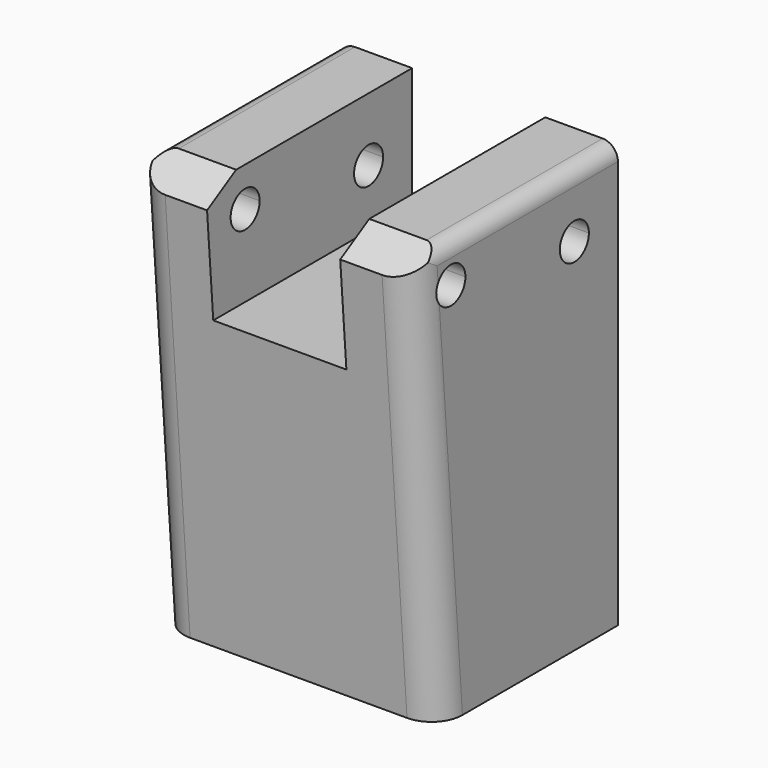
from build123d import *

# Parameters (mm, degrees)
F1_DEPTH     = 46
F3_DEPTH     = 40
F5_DEPTH     = 254
F6_W         = 22
F6_H         = 20
F7_DEPTH     = 1346.2
F8_DEPTH     = 65
F10_DEPTH    = 127
F12_DEPTH    = 254
F14_DEPTH    = 254
F15_T1_DEPTH = 103.8636030304
F15_T3_DEPTH = 103.8636030304
F17_T1_DEPTH = 49.0578822911


# Not quite as in the source:
# - a fillet or chamfer that OpenCascade refuses, or shapes differently, is made with other operations: its cross-section is extruded or revolved along the edge and cut away or added
# - a feature of the source that left no trace in its solid (it failed there, or was rolled back) is left out


with BuildPart() as f1:
    # F0 (on Right) → F1 (new body)
    with BuildSketch(Plane.YZ):
        Polygon((52, 0), (0, 0), (12, -60), (12, -70), (52, -70), align=None)
    extrude(amount=F1_DEPTH)

    # F2 (on face) → F3 (cut)
    with BuildSketch(Plane(origin=(0, 0, -70), x_dir=(1, 0, 0), z_dir=(0, 0, -1))):
        with BuildLine():
            Line((23, -33.3181476), (38, -33.3181476))
            ThreePointArc((38, -33.3181476), (12.3933982822, -22.7115458822), (23, -48.3181476))
            Line((23, -48.3181476), (23, -33.3181476))
        make_face()
        with BuildLine():
            ThreePointArc((23, -48.3181476), (33.6066017178, -43.9247493178), (38, -33.3181476))
            Line((38, -33.3181476), (23, -33.3181476))
            Line((23, -33.3181476), (23, -48.3181476))
        make_face()
    extrude(amount=-F3_DEPTH, mode=Mode.SUBTRACT)

    # F4 (on face) → F5 (cut)
    with BuildSketch(Plane.YZ.offset(46)):
        with BuildLine():
            Line((17.5, -6.5), (20.5, -6.5))
            ThreePointArc((20.5, -6.5), (19.6213203436, -4.3786796564), (17.5, -3.5))
            Line((17.5, -3.5), (17.5, -6.5))
        make_face()
        with BuildLine():
            ThreePointArc((17.5, -3.5), (15.3786796564, -8.6213203436), (20.5, -6.5))
            Line((20.5, -6.5), (17.5, -6.5))
            Line((17.5, -6.5), (17.5, -3.5))
        make_face()
    extrude(amount=-F5_DEPTH, mode=Mode.SUBTRACT)

    # F6 (on face) → F7 (cut)
    with BuildSketch(Plane(origin=(0, 52, 0), x_dir=(-1, 0, 0), z_dir=(0, 1, 0))):
        with Locations((-23, -10)):
            Rectangle(F6_W, F6_H)
    extrude(amount=-F7_DEPTH, mode=Mode.SUBTRACT)

    # F4 (on face) → F8 (cut)
    with BuildSketch(Plane.YZ.offset(46)):
        with BuildLine():
            ThreePointArc((43, -7.5), (40.8786796564, -12.6213203436), (46, -10.5))
            ThreePointArc((46, -10.5), (45.1213203436, -8.3786796564), (43, -7.5))
        make_face()
    extrude(amount=-F8_DEPTH, mode=Mode.SUBTRACT)

    # F9 (on face) → F10 (cut)
    with BuildSketch(Plane.YZ.offset(46)):
        Polygon((1.1435132474, -8.0939428881), (1.6304426827, -8.0939428881), (15.6421177089, 0), (0, 0), align=None)
    extrude(amount=-F10_DEPTH, mode=Mode.SUBTRACT)

    # F11 (on Right) → F12 (cut)
    with BuildSketch(Plane.YZ):
        Polygon((0, -70.3560113907), (14.7977182642, -70.0814500451), (9.3696815893, 0), (0, 0), align=None)
    extrude(amount=F12_DEPTH, mode=Mode.SUBTRACT)

    # F13 (on face) → F14 (cut)
    with BuildSketch(Plane.XY):
        with BuildLine():
            add(Edge.make_bspline(
                [(0, 12.6551715657), (0, 9.9420361221), (2.5992305018, 9.7406599671), (3.9225574583, 9.6255876124)],
                knots=[0, 0, 0, 0, 4.9562925603, 4.9562925603, 4.9562925603, 4.9562925603], degree=3))
            Line((0, 12.6551715657), (0, 9.539283812))
            Line((0, 9.539283812), (3.9225574583, 9.6255876124))
        make_face()
        with BuildLine():
            Line((46, 9.539283812), (46, 12.6551715657))
            add(Edge.make_bspline(
                [(46, 12.6551715657), (46, 9.9420361221), (43.4007694982, 9.7406599671), (42.0774425417, 9.6255876124)],
                knots=[0, 0, 0, 0, 4.9562925603, 4.9562925603, 4.9562925603, 4.9562925603], degree=3))
            Line((42.0774425417, 9.6255876124), (46, 9.539283812))
        make_face()
    extrude(amount=-F14_DEPTH, mode=Mode.SUBTRACT)

    # F15: fillet of radius 5.08 on 2 edges, made by hand

    # F15_s2 → F15_t1 (cut)
    with BuildSketch(Plane(origin=(0, 6.4583208178, -83.3834616235), x_dir=(1, 0, 0), z_dir=(0, -0.0772219774, 0.9970139248))):
        with BuildLine():
            ThreePointArc((0, 14.4217030153), (1.4878975516, 10.8296005669), (5.08, 9.3417030153))
            Line((5.08, 9.3417030153), (0, 9.3417030153))
            Line((0, 9.3417030153), (0, 14.4217030153))
        make_face()
    extrude(amount=F15_T1_DEPTH, mode=Mode.SUBTRACT)

    # F15_s4 → F15_t3 (cut)
    with BuildSketch(Plane(origin=(0, -1.5622319844, 20.169996876), x_dir=(1, 0, 0), z_dir=(0, 0.0772219774, -0.9970139248))):
        with BuildLine():
            ThreePointArc((40.92, -9.3417030153), (44.5121024484, -10.8296005669), (46, -14.4217030153))
            Line((46, -14.4217030153), (46, -9.3417030153))
            Line((46, -9.3417030153), (40.92, -9.3417030153))
        make_face()
    extrude(amount=F15_T3_DEPTH, mode=Mode.SUBTRACT)

    # F17: fillet of radius 2.54 on 2 edges, made by hand

    # F17_s2 → F17_t1 (cut)
    with BuildSketch(Plane.XZ.offset(-58.35)):
        with BuildLine():
            ThreePointArc((2.54, 0), (0.7439487758, -0.7439487758), (0, -2.54))
            Line((0, -2.54), (0, 0))
            Line((0, 0), (2.54, 0))
        make_face()
        with BuildLine():
            ThreePointArc((43.46, 0), (45.2560512242, -0.7439487758), (46, -2.54))
            Line((46, -2.54), (46, 0))
            Line((46, 0), (43.46, 0))
        make_face()
    extrude(amount=F17_T1_DEPTH, mode=Mode.SUBTRACT)


solid = f1.part
